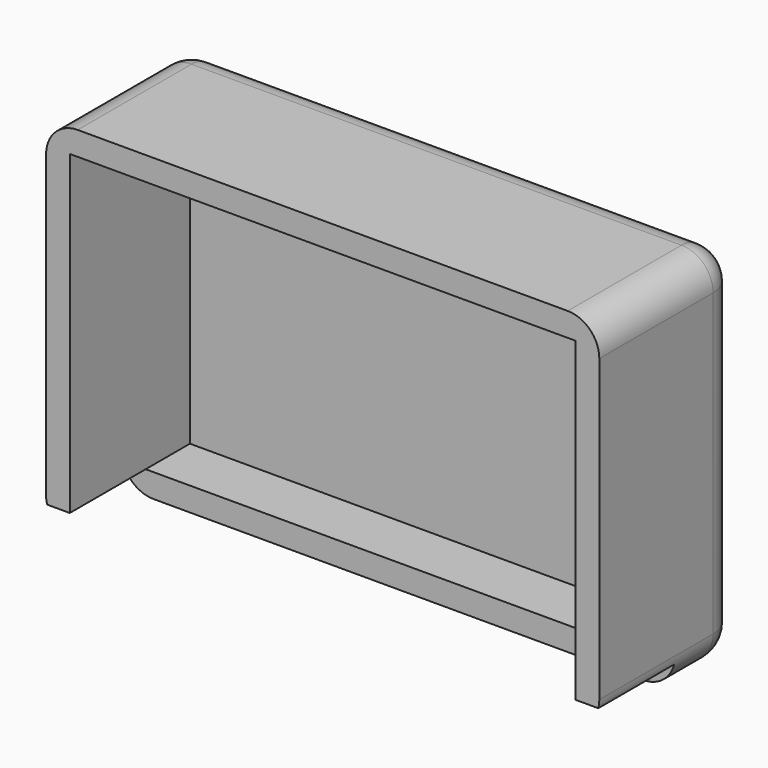
from build123d import *

# Parameters (mm, degrees)
F0_W         = 32
F0_H         = 20
F1_DEPTH     = 1.5
F2_DEPTH     = 11
F3_DEPTH     = 5
F4_R         = 2
F5_T1_DEPTH  = 15
F5_S5_W      = 2.04
F5_S5_H      = 2.04
F5_T6_DEPTH  = 2.04
F5_S11_W     = 2.04
F5_S11_H     = 2.04
F5_T12_DEPTH = 2.04


# Not quite as in the source:
# - a fillet or chamfer that OpenCascade refuses, or shapes differently, is made with other operations: its cross-section is extruded or revolved along the edge and cut away or added


with BuildPart() as f1:
    # F0 (on Front) → F1 (new body)
    with BuildSketch(Plane.XZ):
        with Locations((0.460526906, 4.9254382253)):
            Rectangle(F0_W, F0_H)
    extrude(amount=F1_DEPTH)

    # F0 (on Front) → F2 (join)
    with BuildSketch(Plane.XZ):
        Polygon((-15.539473094, -5.0745617747), (-15.539473094, 14.9254382253), (16.460526906, 14.9254382253), (16.460526906, -5.0745617747), (17.960526906, -5.0745617747), (17.960526906, 16.4254382253), (-17.039473094, 16.4254382253), (-17.039473094, -5.0745617747), align=None)
    extrude(amount=F2_DEPTH)

    # F0 (on Front) → F3 (join)
    with BuildSketch(Plane.XZ):
        Polygon((16.460526906, -5.0745617747), (-15.539473094, -5.0745617747), (-17.039473094, -5.0745617747), (-17.039473094, -6.5745617747), (17.960526906, -6.5745617747), (17.960526906, -5.0745617747), align=None)
    extrude(amount=F3_DEPTH)

    # F4
    f4_edges = [f1.edges().sort_by_distance(p)[0] for p in [
        (17.960527, 0, 4.925438),
        (0.460527, 0, 16.425438),
        (-17.039473, 0, 4.925438),
        (0.460527, 0, -6.574562),
        (17.960527, -5.5, 16.425438),
        (-17.039473, -5.5, 16.425438),
    ]]
    fillet(f4_edges, radius=F4_R)

    # F5: fillet of radius 2 on 2 edges, made by hand

    # F5_s2 → F5_t1 (cut)
    with BuildSketch(Plane.XZ.offset(2)):
        with BuildLine():
            ThreePointArc((-17.039473094, -4.5745617747), (-16.4536866564, -5.9887753371), (-15.039473094, -6.5745617747))
            Line((-15.039473094, -6.5745617747), (-15.039473094, -6.6145617747))
            Line((-15.039473094, -6.6145617747), (-17.079473094, -6.6145617747))
            Line((-17.079473094, -6.6145617747), (-17.079473094, -4.5745617747))
            Line((-17.079473094, -4.5745617747), (-17.039473094, -4.5745617747))
        make_face()
        with BuildLine():
            ThreePointArc((15.960526906, -6.5745617747), (17.3747404683, -5.9887753371), (17.960526906, -4.5745617747))
            Line((17.960526906, -4.5745617747), (18.000526906, -4.5745617747))
            Line((18.000526906, -4.5745617747), (18.000526906, -6.6145617747))
            Line((18.000526906, -6.6145617747), (15.960526906, -6.6145617747))
            Line((15.960526906, -6.6145617747), (15.960526906, -6.5745617747))
        make_face()
    extrude(amount=F5_T1_DEPTH, mode=Mode.SUBTRACT)


with BuildPart() as f5_tool4:
    # F5_s5 → F5_t6 (new body)
    with BuildSketch(Plane.XY.offset(-4.5745617747)):
        with Locations((16.980526906, -0.98)):
            Rectangle(F5_S5_W, F5_S5_H)
    extrude(amount=-F5_T6_DEPTH)

    # F5_s7 → F5_t8 (revolve, cut)
    with BuildSketch(Plane(origin=(15.960526906, -2, -4.5745617747), x_dir=(-0.7071067812, -0.7071067812, 0), z_dir=(0.7071067812, -0.7071067812, 0))):
        with BuildLine():
            ThreePointArc((0, -2), (2, 0), (0, 2))
            Line((0, 2), (0, -2))
        make_face()
    revolve(axis=Axis((15.960526906, -2, -4.5745617747), (0, 0, -1)), mode=Mode.SUBTRACT)


with BuildPart() as f1_1:
    add(f1.part)

    # F5_t3: cut F5_tool4
    add(f5_tool4.part, mode=Mode.SUBTRACT)


with BuildPart() as f5_tool10:
    # F5_s11 → F5_t12 (new body)
    with BuildSketch(Plane.YZ.offset(-15.039473094)):
        with Locations((-0.98, -5.5945617747)):
            Rectangle(F5_S11_W, F5_S11_H)
    extrude(amount=-F5_T12_DEPTH)

    # F5_s13 → F5_t14 (revolve, cut)
    with BuildSketch(Plane(origin=(-15.039473094, -2, -4.5745617747), x_dir=(0, -0.7071067812, 0.7071067812), z_dir=(0, -0.7071067812, -0.7071067812))):
        with BuildLine():
            ThreePointArc((0, -2), (2, 0), (0, 2))
            Line((0, 2), (0, -2))
        make_face()
    revolve(axis=Axis((-15.039473094, -2, -4.5745617747), (-1, 0, 0)), mode=Mode.SUBTRACT)


with BuildPart() as f1_2:
    add(f1_1.part)

    # F5_t9: cut F5_tool10
    add(f5_tool10.part, mode=Mode.SUBTRACT)


solid = f1_2.part
